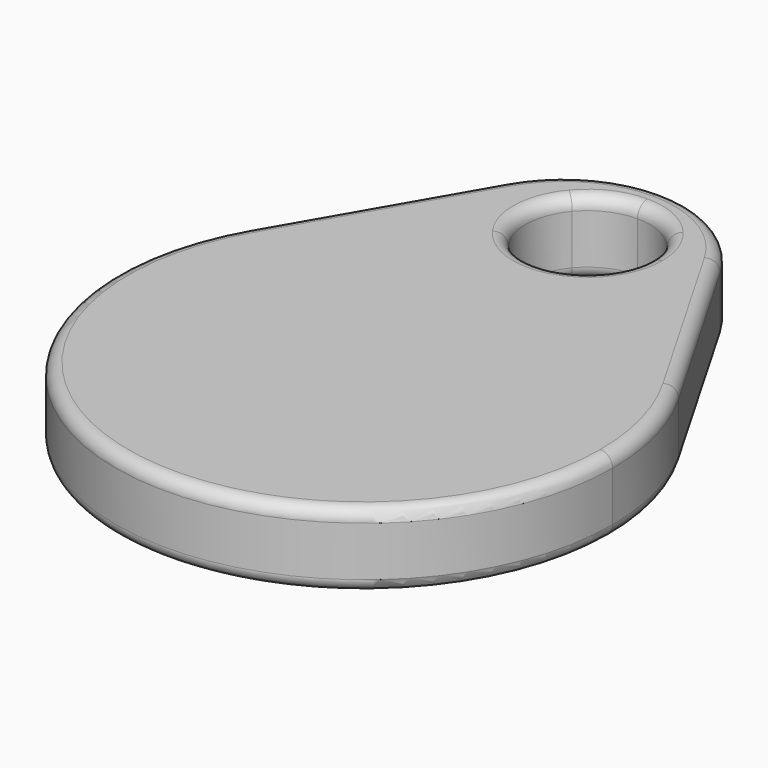
from build123d import *

# Parameters (mm, degrees)
F1_DEPTH = 3
F2_R     = 0.5


with BuildPart() as f1:
    # F0 (on Top) → F1 (new body)
    with BuildSketch(Plane.XY):
        with BuildLine():
            ThreePointArc((-8.6602540378, 5), (-2.588190451, -9.6592582629), (10, 0))
            ThreePointArc((10, 0), (9.6592582629, 2.588190451), (8.6602540378, 5))
            ThreePointArc((8.6602540378, 5), (7.0062926922, 7.1352549156), (4.8412291828, 8.75))
            ThreePointArc((4.8412291828, 8.75), (0, 5), (-4.8412291828, 8.75))
            ThreePointArc((-4.8412291828, 8.75), (-7.0062926922, 7.1352549156), (-8.6602540378, 5))
        make_face()
        with BuildLine():
            Line((-4.3301270189, 12.5), (-8.6602540378, 5))
            ThreePointArc((-8.6602540378, 5), (-7.0062926922, 7.1352549156), (-4.8412291828, 8.75))
            ThreePointArc((-4.8412291828, 8.75), (-4.9541970736, 10.6752268918), (-4.3301270189, 12.5))
        make_face()
        with BuildLine():
            ThreePointArc((-4.8412291828, 8.75), (0, 5), (4.8412291828, 8.75))
            ThreePointArc((4.8412291828, 8.75), (3.4751568493, 9.3767416981), (2.0305821552, 9.7916666667))
            ThreePointArc((2.0305821552, 9.7916666667), (0, 8.75), (-2.0305821552, 9.7916666667))
            ThreePointArc((-2.0305821552, 9.7916666667), (-3.4751568493, 9.3767416981), (-4.8412291828, 8.75))
        make_face()
        with BuildLine():
            ThreePointArc((2.0305821552, 9.7916666667), (3.4751568493, 9.3767416981), (4.8412291828, 8.75))
            ThreePointArc((4.8412291828, 8.75), (4.9601484813, 9.3699785376), (5, 10))
            ThreePointArc((5, 10), (4.8296291314, 11.2940952255), (4.3301270189, 12.5))
            ThreePointArc((4.3301270189, 12.5), (2.5, 14.3301270189), (0, 15))
            Line((0, 15), (0, 13.75))
            ThreePointArc((0, 13.75), (1.0557382883, 13.5161457735), (1.9139654879, 12.8583333333))
            ThreePointArc((1.9139654879, 12.8583333333), (2.3489267464, 12.1058873408), (2.5, 11.25))
            ThreePointArc((2.5, 11.25), (2.3797537045, 10.4839893564), (2.0305821552, 9.7916666667))
        make_face()
        with BuildLine():
            ThreePointArc((4.8412291828, 8.75), (7.0062926922, 7.1352549156), (8.6602540378, 5))
            Line((8.6602540378, 5), (4.3301270189, 12.5))
            ThreePointArc((4.3301270189, 12.5), (4.8296291314, 11.2940952255), (5, 10))
            ThreePointArc((5, 10), (4.9601484813, 9.3699785376), (4.8412291828, 8.75))
        make_face()
        with BuildLine():
            ThreePointArc((-4.3301270189, 12.5), (-4.9541970736, 10.6752268918), (-4.8412291828, 8.75))
            ThreePointArc((-4.8412291828, 8.75), (-3.4751568493, 9.3767416981), (-2.0305821552, 9.7916666667))
            ThreePointArc((-2.0305821552, 9.7916666667), (-2.4981943756, 11.3449992725), (-1.9139654879, 12.8583333333))
            ThreePointArc((-1.9139654879, 12.8583333333), (-1.0557382883, 13.5161457735), (0, 13.75))
            Line((0, 13.75), (0, 15))
            ThreePointArc((0, 15), (-2.5, 14.3301270189), (-4.3301270189, 12.5))
        make_face()
    extrude(amount=F1_DEPTH)

    # F2
    f2_edges = [f1.edges().sort_by_distance(p)[0] for p in [
        (6.495191, 8.75, 3),
        (0, 15, 3),
        (0, 15, 0),
        (6.495191, 8.75, 0),
        (0, -10, 0),
        (0, -10, 3),
        (-6.495191, 8.75, 3),
        (2.030582, 12.708333, 3),
        (2.030582, 12.708333, 0),
        (-6.495191, 8.75, 0),
    ]]
    fillet(f2_edges, radius=F2_R)


solid = f1.part
